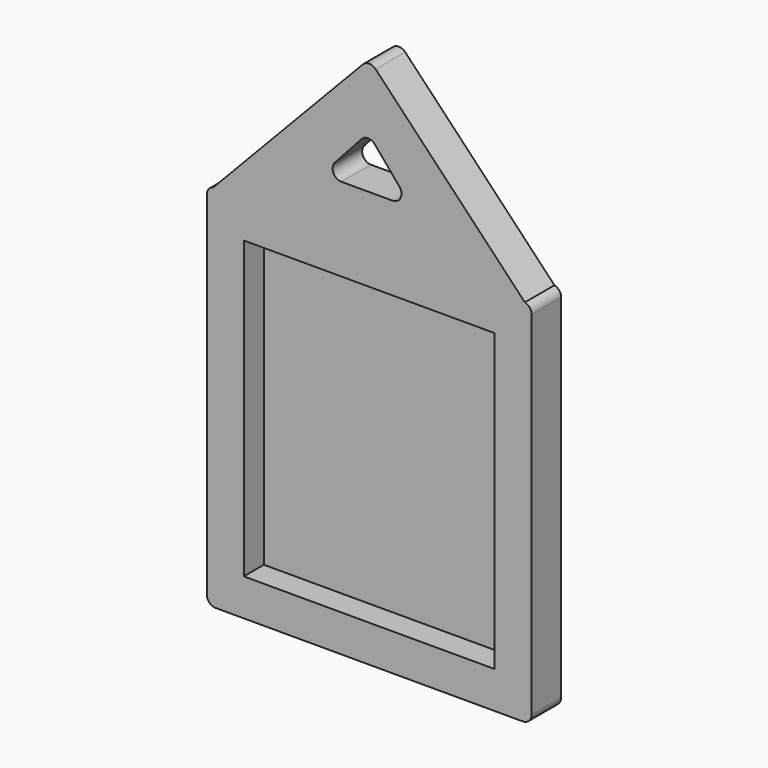
from build123d import *

# Parameters (mm, degrees)
F1_DEPTH     = 6.35
F2_W         = 43.0978981023
F2_H         = 50.8
F3_DEPTH     = 4.318
F5_DEPTH     = 6.35
F7_DEPTH     = 6.351
F8_T1_DEPTH  = 6.35
F8_T3_DEPTH  = 6.35
F8_T5_DEPTH  = 6.35
F8_T7_DEPTH  = 13.7467402192
F8_T9_DEPTH  = 14.3479140779
F8_T11_DEPTH = 13.97
F8_T13_DEPTH = 13.97
F8_T15_DEPTH = 13.724225926


# Not quite as in the source:
# - a fillet or chamfer that OpenCascade refuses, or shapes differently, is made with other operations: its cross-section is extruded or revolved along the edge and cut away or added


with BuildPart() as f1:
    # F0 (on Front) → F1 (new body)
    with BuildSketch(Plane.XZ):
        Polygon((-40.601760045, 44.2037712147), (-40.601760045, 20.0136204353), (-40.601760045, -19.2962287853), (-31.9894673416, -19.2962287853), (6.5923849878, -19.2962287853), (15.1961380572, -19.2962287853), (15.1961380572, 20.0136204353), (15.1961380572, 44.2037712147), align=None)
    extrude(amount=F1_DEPTH)

    # F2 (on face) → F3 (cut, through all)
    with BuildSketch(Plane.XZ.offset(6.35)):
        with Locations((-12.7028109939, 12.4537712147)):
            Rectangle(F2_W, F2_H)
    extrude(amount=-F3_DEPTH, mode=Mode.SUBTRACT)

    # F4 (on Front) → F5 (join, through all)
    with BuildSketch(Plane.XZ):
        Polygon((-12.7028109939, 72.2804571797), (-39.4616971228, 44.2037712147), (14.0383420512, 44.2037712147), align=None)
    extrude(amount=F5_DEPTH)

    # F6 (on Front) → F7 (cut, through all)
    with BuildSketch(Plane.XZ):
        Polygon((-5.3985980339, 52.1819666028), (-12.8735816106, 61.0412061214), (-20.9022667259, 52.1819666028), align=None)
    extrude(amount=F7_DEPTH, mode=Mode.SUBTRACT)

    # F8: fillet of radius 1.524 on 8 edges, made by hand

    # F8_s2 → F8_t1 (join)
    with BuildSketch(Plane.XZ):
        with BuildLine():
            ThreePointArc((-11.7497792539, 59.7092922586), (-12.8875838111, 60.2502701687), (-14.0438236179, 59.7499044838))
            Line((-14.0438236179, 59.7499044838), (-12.8735816106, 61.0412061214))
            Line((-12.8735816106, 61.0412061214), (-11.7497792539, 59.7092922586))
        make_face()
    extrude(amount=F8_T1_DEPTH)

    # F8_s4 → F8_t3 (join)
    with BuildSketch(Plane.XZ):
        with BuildLine():
            ThreePointArc((-7.5136965339, 54.688749932), (-7.2963881401, 53.0637772981), (-8.6784767396, 52.1819666028))
            Line((-8.6784767396, 52.1819666028), (-5.3985980339, 52.1819666028))
            Line((-5.3985980339, 52.1819666028), (-7.5136965339, 54.688749932))
        make_face()
    extrude(amount=F8_T3_DEPTH)

    # F8_s6 → F8_t5 (join)
    with BuildSketch(Plane.XZ):
        with BuildLine():
            ThreePointArc((-17.4644255473, 52.1819666028), (-18.8576647272, 53.0883416458), (-18.5936897056, 54.7293621572))
            Line((-18.5936897056, 54.7293621572), (-20.9022667259, 52.1819666028))
            Line((-20.9022667259, 52.1819666028), (-17.4644255473, 52.1819666028))
        make_face()
    extrude(amount=F8_T5_DEPTH)

    # F8_s8 → F8_t7 (cut)
    with BuildSketch(Plane.XZ.offset(-3.6983701096)):
        with BuildLine():
            ThreePointArc((14.0383420512, 44.2037712147), (14.8722778172, 43.6636997843), (15.1961380572, 42.7244231708))
            Line((15.1961380572, 42.7244231708), (15.1961380572, 44.2037712147))
            Line((15.1961380572, 44.2037712147), (14.0383420512, 44.2037712147))
        make_face()
    extrude(amount=F8_T7_DEPTH, mode=Mode.SUBTRACT)

    # F8_s10 → F8_t9 (cut)
    with BuildSketch(Plane.XZ.offset(-3.9989570389)):
        with BuildLine():
            ThreePointArc((-11.5996190182, 71.1221685073), (-12.7029244443, 71.5951040748), (-13.8063863853, 71.122533806))
            Line((-13.8063863853, 71.122533806), (-12.7028109939, 72.2804571797))
            Line((-12.7028109939, 72.2804571797), (-11.5996190182, 71.1221685073))
        make_face()
    extrude(amount=F8_T9_DEPTH, mode=Mode.SUBTRACT)

    # F8_s12 → F8_t11 (cut)
    with BuildSketch(Plane.XZ.offset(-3.81)):
        with BuildLine():
            ThreePointArc((15.1961380572, -17.7722287853), (14.7497687918, -18.8498595199), (13.6721380572, -19.2962287853))
            Line((13.6721380572, -19.2962287853), (15.1961380572, -19.2962287853))
            Line((15.1961380572, -19.2962287853), (15.1961380572, -17.7722287853))
        make_face()
    extrude(amount=F8_T11_DEPTH, mode=Mode.SUBTRACT)

    # F8_s14 → F8_t13 (cut)
    with BuildSketch(Plane.XZ.offset(-3.81)):
        with BuildLine():
            ThreePointArc((-39.077760045, -19.2962287853), (-40.1553907795, -18.8498595199), (-40.601760045, -17.7722287853))
            Line((-40.601760045, -17.7722287853), (-40.601760045, -19.2962287853))
            Line((-40.601760045, -19.2962287853), (-39.077760045, -19.2962287853))
        make_face()
    extrude(amount=F8_T13_DEPTH, mode=Mode.SUBTRACT)

    # F8_s16 → F8_t15 (cut)
    with BuildSketch(Plane.XZ.offset(-3.687112963)):
        with BuildLine():
            ThreePointArc((-40.601760045, 42.7289260295), (-40.2835162614, 43.6609817932), (-39.4616971228, 44.2037712147))
            Line((-39.4616971228, 44.2037712147), (-40.601760045, 44.2037712147))
            Line((-40.601760045, 44.2037712147), (-40.601760045, 42.7289260295))
        make_face()
    extrude(amount=F8_T15_DEPTH, mode=Mode.SUBTRACT)


solid = f1.part
